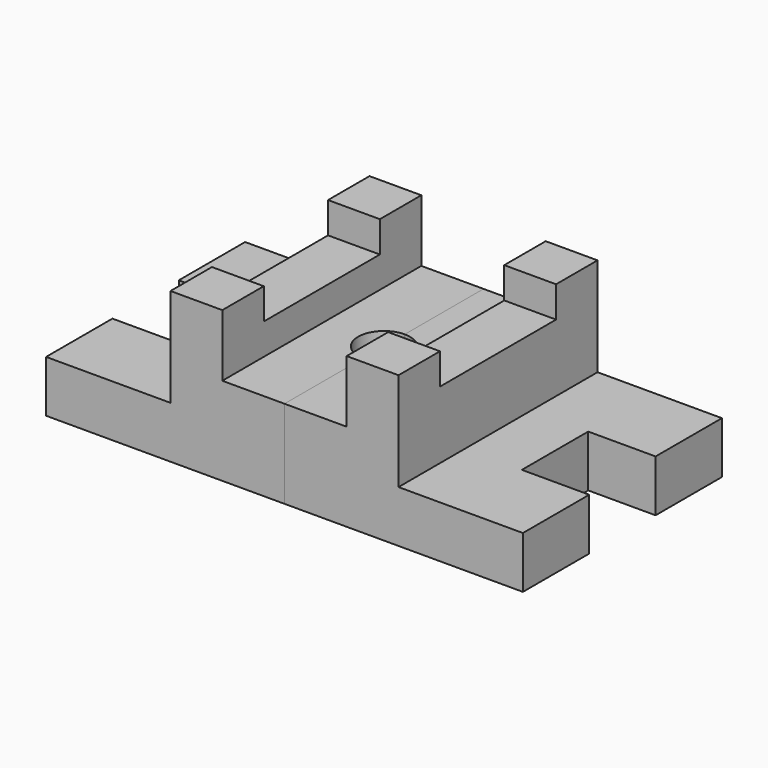
from build123d import *
from build123d import SkipClean  # not in build123d's __all__

# Parameters (mm, degrees)
F1_DEPTH = 31.75
F2_DEPTH = 53.975
F3_DEPTH = 73.025
F0_W     = 31.75
F0_H     = 31.75
F4_DEPTH = 92.075
F5_DEPTH = 73.025


with BuildPart() as f1:
    # F0 (on Top) → F1 (new body)
    with BuildSketch(Plane.XY):
        Polygon((108.4912913322, 117.0880892358), (32.2912913322, 117.0880892358), (32.2912913322, 85.3380892358), (32.2912913322, 15.4880892358), (32.2912913322, -3.5619107642), (32.2912913322, -16.2619107642), (32.2912913322, -35.3119107642), (108.4912913322, -35.3119107642), (108.4912913322, 15.4880892358), (67.2162913322, 15.4880892358), (67.2162913322, 66.2880892358), (108.4912913322, 66.2880892358), align=None)
    extrude(amount=F1_DEPTH)



with BuildPart() as f2:
    # F0 (on Top) → F2 (new body)
    with BuildSketch(Plane.XY):
        with BuildLine():
            Line((0.5412913322, 117.0880892358), (-37.5587086678, 117.0880892358))
            Line((-37.5587086678, 117.0880892358), (-37.5587086678, 56.7630892358))
            ThreePointArc((-37.5587086678, 56.7630892358), (-21.6837086678, 40.8880892358), (-37.5587086678, 25.0130892358))
            Line((-37.5587086678, 25.0130892358), (-37.5587086678, -35.3119107642))
            Line((-37.5587086678, -35.3119107642), (0.5412913322, -35.3119107642))
            Line((0.5412913322, -35.3119107642), (0.5412913322, -3.5619107642))
            Line((0.5412913322, -3.5619107642), (0.5412913322, 15.4880892358))
            Line((0.5412913322, 15.4880892358), (0.5412913322, 85.3380892358))
            Line((0.5412913322, 85.3380892358), (0.5412913322, 117.0880892358))
        make_face()
    extrude(amount=F2_DEPTH)


with BuildPart() as f1_1:
    add(f1.part, clean=False)

    add(f2.part)  # F3 merges F2
    # F0 (on Top) → F3 (join)
    with BuildSketch(Plane.XY):
        Polygon((32.2912913322, 85.3380892358), (0.5412913322, 85.3380892358), (0.5412913322, 15.4880892358), (0.5412913322, -3.5619107642), (32.2912913322, -3.5619107642), (32.2912913322, 15.4880892358), align=None)
    extrude(amount=F3_DEPTH)

    # F0 (on Top) → F4 (join)
    with BuildSketch(Plane.XY):
        Polygon((32.2912913322, -3.5619107642), (0.5412913322, -3.5619107642), (0.5412913322, -35.3119107642), (32.2912913322, -35.3119107642), (32.2912913322, -16.2619107642), align=None)
        with Locations((16.4162913322, 101.2130892358)):
            Rectangle(F0_W, F0_H)
    extrude(amount=F4_DEPTH)

    # F0 (on Top) → F5 (join)
    with BuildSketch(Plane.XY):
        Polygon((32.2912913322, 85.3380892358), (0.5412913322, 85.3380892358), (0.5412913322, 15.4880892358), (0.5412913322, -3.5619107642), (32.2912913322, -3.5619107642), (32.2912913322, 15.4880892358), align=None)
    extrude(amount=F5_DEPTH)

    # F6: F1 across face


with BuildPart() as f1_2:
    add(f1_1.part, clean=False)
    with SkipClean():  # cleaning this boolean's faces spoils the solid; the shape is the same uncleaned
        add(f1_1.part.mirror(Plane(origin=(-37.5587086678, 86.9255892358, 26.9875), x_dir=(0, -1, 0), z_dir=(-1, 0, 0))), clean=False)


solid = f1_2.part
